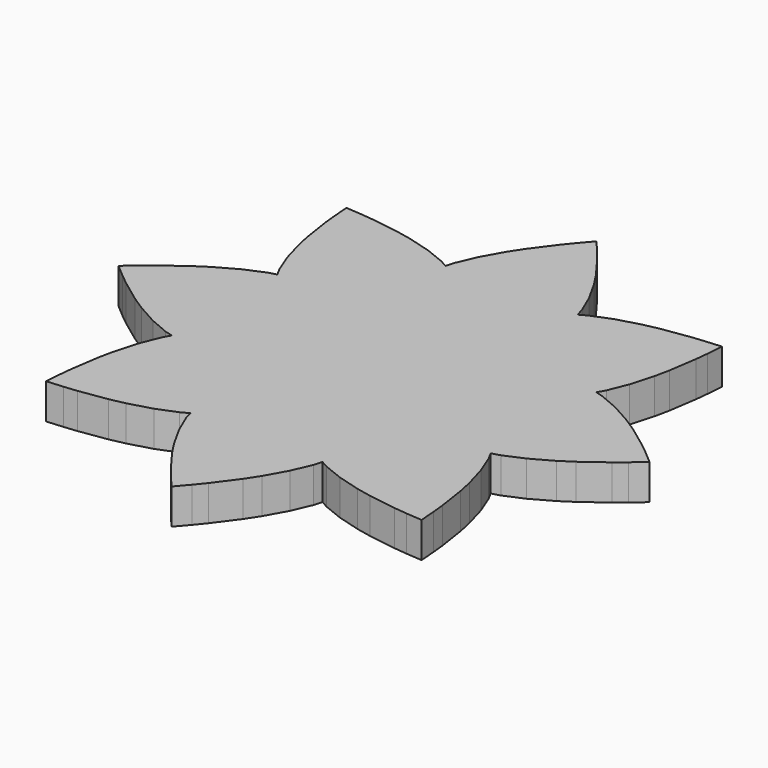
from build123d import *

# Parameters (mm, degrees)
F1_DEPTH = 6


with BuildPart() as f1:
    # F0 (on Top) → F1 (new body)
    with BuildSketch(Plane.XY):
        with BuildLine():
            ThreePointArc((11.0582894347, -1.2164948741), (11.1083098391, -0.6091613247), (11.125, 0))
            ThreePointArc((11.125, 0), (11.1083098391, 0.6091613247), (11.0582894347, 1.2164948741))
            Line((11.0582894347, 1.2164948741), (5.1512120865, 0.50045829))
            Line((5.1512120865, 0.50045829), (0, 0))
            Line((0, 0), (5.1512120865, -0.50045829))
            Line((5.1512120865, -0.50045829), (11.0582894347, -1.2164948741))
        make_face()
        with BuildLine():
            ThreePointArc((11.0582894347, 1.2164948741), (11.1083098391, 0.6091613247), (11.125, 0))
            ThreePointArc((11.125, 0), (11.1083098391, -0.6091613247), (11.0582894347, -1.2164948741))
            Line((11.0582894347, -1.2164948741), (14.5342076496, -1.8604729178))
            ThreePointArc((14.5342076496, -1.8604729178), (14.6231219501, -0.9321244087), (14.6528001242, 0))
            ThreePointArc((14.6528001242, 0), (14.6231219501, 0.9321244087), (14.5342076496, 1.8604729178))
            Line((14.5342076496, 1.8604729178), (11.0582894347, 1.2164948741))
        make_face()
        with BuildLine():
            Line((5.1512120865, 0.50045829), (11.0582894347, 1.2164948741))
            ThreePointArc((11.0582894347, 1.2164948741), (10.2781597992, 4.2573531851), (8.6795832223, 6.9591996729))
            Line((8.6795832223, 6.9591996729), (3.9963344483, 3.2885795472))
            Line((3.9963344483, 3.2885795472), (0, 0))
            Line((0, 0), (5.1512120865, 0.50045829))
        make_face()
        with BuildLine():
            ThreePointArc((8.6795832223, 6.9591996729), (10.2781597992, 4.2573531851), (11.0582894347, 1.2164948741))
            Line((11.0582894347, 1.2164948741), (14.5342076496, 1.8604729178))
            ThreePointArc((14.5342076496, 1.8604729178), (13.5374221288, 5.6073838453), (11.5927898046, 8.9616837719))
            Line((11.5927898046, 8.9616837719), (8.6795832223, 6.9591996729))
        make_face()
        with BuildLine():
            Line((14.5342076496, -1.8604729178), (11.0582894347, -1.2164948741))
            ThreePointArc((11.0582894347, -1.2164948741), (10.2781597992, -4.2573531851), (8.6795832223, -6.9591996729))
            Line((8.6795832223, -6.9591996729), (11.5927898046, -8.9616837719))
            ThreePointArc((11.5927898046, -8.9616837719), (13.5374221288, -5.6073838453), (14.5342076496, -1.8604729178))
        make_face()
        with BuildLine():
            ThreePointArc((8.6795832223, -6.9591996729), (10.2781597992, -4.2573531851), (11.0582894347, -1.2164948741))
            Line((11.0582894347, -1.2164948741), (5.1512120865, -0.50045829))
            Line((5.1512120865, -0.50045829), (0, 0))
            Line((0, 0), (3.9963344483, -3.2885795472))
            Line((3.9963344483, -3.2885795472), (8.6795832223, -6.9591996729))
        make_face()
        with BuildLine():
            Line((3.9963344483, 3.2885795472), (8.6795832223, 6.9591996729))
            ThreePointArc((8.6795832223, 6.9591996729), (7.8665629407, 7.8665629407), (6.9591996729, 8.6795832223))
            Line((6.9591996729, 8.6795832223), (3.2885795472, 3.9963344483))
            Line((3.2885795472, 3.9963344483), (0, 0))
            Line((0, 0), (3.9963344483, 3.2885795472))
        make_face()
        with BuildLine():
            ThreePointArc((6.9591996729, 8.6795832223), (7.8665629407, 7.8665629407), (8.6795832223, 6.9591996729))
            Line((8.6795832223, 6.9591996729), (11.5927898046, 8.9616837719))
            ThreePointArc((11.5927898046, 8.9616837719), (10.3610943312, 10.3610943312), (8.9616837719, 11.5927898046))
            Line((8.9616837719, 11.5927898046), (6.9591996729, 8.6795832223))
        make_face()
        with BuildLine():
            Line((15.430184363, 2.1339611713), (14.5342076496, 1.8604729178))
            ThreePointArc((14.5342076496, 1.8604729178), (14.6231219501, 0.9321244087), (14.6528001242, 0))
            ThreePointArc((14.6528001242, 0), (14.6231219501, -0.9321244087), (14.5342076496, -1.8604729178))
            Line((14.5342076496, -1.8604729178), (15.430184363, -2.1339611713))
            ThreePointArc((15.430184363, -2.1339611713), (15.124443045, 0), (15.430184363, 2.1339611713))
        make_face()
        with BuildLine():
            ThreePointArc((11.5927898046, 8.9616837719), (13.5374221288, 5.6073838453), (14.5342076496, 1.8604729178))
            Line((14.5342076496, 1.8604729178), (15.430184363, 2.1339611713))
            ThreePointArc((15.430184363, 2.1339611713), (18.8444497658, 6.5349561707), (24.3428657322, 7.4256789592))
            Line((24.3428657322, 7.4256789592), (26.2042805414, 9.6967201996))
            Line((26.2042805414, 9.6967201996), (27.0298449885, 11.1961283831))
            Line((27.0298449885, 11.1961283831), (25.3858410754, 11.6726078585))
            Line((25.3858410754, 11.6726078585), (22.4637533797, 11.9622574858))
            ThreePointArc((22.4637533797, 11.9622574858), (17.9459500402, 8.704126394), (12.419726413, 9.401849583))
            Line((12.419726413, 9.401849583), (11.5927898046, 8.9616837719))
        make_face()
        with BuildLine():
            Line((11.5927898046, -8.9616837719), (8.6795832223, -6.9591996729))
            ThreePointArc((8.6795832223, -6.9591996729), (7.8665629407, -7.8665629407), (6.9591996729, -8.6795832223))
            Line((6.9591996729, -8.6795832223), (8.9616837719, -11.5927898046))
            ThreePointArc((8.9616837719, -11.5927898046), (10.3610943312, -10.3610943312), (11.5927898046, -8.9616837719))
        make_face()
        with BuildLine():
            ThreePointArc((6.9591996729, -8.6795832223), (7.8665629407, -7.8665629407), (8.6795832223, -6.9591996729))
            Line((8.6795832223, -6.9591996729), (3.9963344483, -3.2885795472))
            Line((3.9963344483, -3.2885795472), (0, 0))
            Line((0, 0), (3.2885795472, -3.9963344483))
            Line((3.2885795472, -3.9963344483), (6.9591996729, -8.6795832223))
        make_face()
        with BuildLine():
            Line((15.430184363, -2.1339611713), (14.5342076496, -1.8604729178))
            ThreePointArc((14.5342076496, -1.8604729178), (13.5374221288, -5.6073838453), (11.5927898046, -8.9616837719))
            Line((11.5927898046, -8.9616837719), (12.419726413, -9.401849583))
            ThreePointArc((12.419726413, -9.401849583), (17.9459500402, -8.704126394), (22.4637533797, -11.9622574858))
            Line((22.4637533797, -11.9622574858), (25.3858410754, -11.6726078585))
            Line((25.3858410754, -11.6726078585), (27.0298449885, -11.1961283831))
            Line((27.0298449885, -11.1961283831), (26.2042805414, -9.6967201996))
            Line((26.2042805414, -9.6967201996), (24.3428657322, -7.4256789592))
            ThreePointArc((24.3428657322, -7.4256789592), (18.8444497658, -6.5349561707), (15.430184363, -2.1339611713))
        make_face()
        with BuildLine():
            Line((3.2885795472, 3.9963344483), (6.9591996729, 8.6795832223))
            ThreePointArc((6.9591996729, 8.6795832223), (4.2573531851, 10.2781597992), (1.2164948741, 11.0582894347))
            Line((1.2164948741, 11.0582894347), (0.50045829, 5.1512120865))
            Line((0.50045829, 5.1512120865), (0, 0))
            Line((0, 0), (3.2885795472, 3.9963344483))
        make_face()
        with BuildLine():
            ThreePointArc((1.2164948741, 11.0582894347), (4.2573531851, 10.2781597992), (6.9591996729, 8.6795832223))
            Line((6.9591996729, 8.6795832223), (8.9616837719, 11.5927898046))
            ThreePointArc((8.9616837719, 11.5927898046), (5.6073838453, 13.5374221288), (1.8604729178, 14.5342076496))
            Line((1.8604729178, 14.5342076496), (1.2164948741, 11.0582894347))
        make_face()
        with BuildLine():
            ThreePointArc((8.9616837719, 11.5927898046), (10.3610943312, 10.3610943312), (11.5927898046, 8.9616837719))
            Line((11.5927898046, 8.9616837719), (12.419726413, 9.401849583))
            ThreePointArc((12.419726413, 9.401849583), (10.6945962388, 10.6945962388), (9.401849583, 12.419726413))
            Line((9.401849583, 12.419726413), (8.9616837719, 11.5927898046))
        make_face()
        with BuildLine():
            Line((-0.50045829, 5.1512120865), (0, 0))
            Line((0, 0), (0.50045829, 5.1512120865))
            Line((0.50045829, 5.1512120865), (1.2164948741, 11.0582894347))
            ThreePointArc((1.2164948741, 11.0582894347), (0, 11.125), (-1.2164948741, 11.0582894347))
            Line((-1.2164948741, 11.0582894347), (-0.50045829, 5.1512120865))
        make_face()
        with BuildLine():
            Line((-3.9963344483, 3.2885795472), (0, 0))
            Line((0, 0), (-3.2885795472, 3.9963344483))
            Line((-3.2885795472, 3.9963344483), (-6.9591996729, 8.6795832223))
            ThreePointArc((-6.9591996729, 8.6795832223), (-7.8665629407, 7.8665629407), (-8.6795832223, 6.9591996729))
            Line((-8.6795832223, 6.9591996729), (-3.9963344483, 3.2885795472))
        make_face()
        with BuildLine():
            Line((-5.1512120865, -0.50045829), (0, 0))
            Line((0, 0), (-5.1512120865, 0.50045829))
            Line((-5.1512120865, 0.50045829), (-11.0582894347, 1.2164948741))
            ThreePointArc((-11.0582894347, 1.2164948741), (-11.125, 0), (-11.0582894347, -1.2164948741))
            Line((-11.0582894347, -1.2164948741), (-5.1512120865, -0.50045829))
        make_face()
        with BuildLine():
            Line((-3.2885795472, 3.9963344483), (0, 0))
            Line((0, 0), (-0.50045829, 5.1512120865))
            Line((-0.50045829, 5.1512120865), (-1.2164948741, 11.0582894347))
            ThreePointArc((-1.2164948741, 11.0582894347), (-4.2573531851, 10.2781597992), (-6.9591996729, 8.6795832223))
            Line((-6.9591996729, 8.6795832223), (-3.2885795472, 3.9963344483))
        make_face()
        with BuildLine():
            Line((-3.2885795472, -3.9963344483), (0, 0))
            Line((0, 0), (-3.9963344483, -3.2885795472))
            Line((-3.9963344483, -3.2885795472), (-8.6795832223, -6.9591996729))
            ThreePointArc((-8.6795832223, -6.9591996729), (-7.8665629407, -7.8665629407), (-6.9591996729, -8.6795832223))
            Line((-6.9591996729, -8.6795832223), (-3.2885795472, -3.9963344483))
        make_face()
        with BuildLine():
            Line((-5.1512120865, 0.50045829), (0, 0))
            Line((0, 0), (-3.9963344483, 3.2885795472))
            Line((-3.9963344483, 3.2885795472), (-8.6795832223, 6.9591996729))
            ThreePointArc((-8.6795832223, 6.9591996729), (-10.2781597992, 4.2573531851), (-11.0582894347, 1.2164948741))
            Line((-11.0582894347, 1.2164948741), (-5.1512120865, 0.50045829))
        make_face()
        with BuildLine():
            Line((0.50045829, -5.1512120865), (0, 0))
            Line((0, 0), (-0.50045829, -5.1512120865))
            Line((-0.50045829, -5.1512120865), (-1.2164948741, -11.0582894347))
            ThreePointArc((-1.2164948741, -11.0582894347), (0, -11.125), (1.2164948741, -11.0582894347))
            Line((1.2164948741, -11.0582894347), (0.50045829, -5.1512120865))
        make_face()
        with BuildLine():
            Line((-3.9963344483, -3.2885795472), (0, 0))
            Line((0, 0), (-5.1512120865, -0.50045829))
            Line((-5.1512120865, -0.50045829), (-11.0582894347, -1.2164948741))
            ThreePointArc((-11.0582894347, -1.2164948741), (-10.2781597992, -4.2573531851), (-8.6795832223, -6.9591996729))
            Line((-8.6795832223, -6.9591996729), (-3.9963344483, -3.2885795472))
        make_face()
        with BuildLine():
            Line((-0.50045829, -5.1512120865), (0, 0))
            Line((0, 0), (-3.2885795472, -3.9963344483))
            Line((-3.2885795472, -3.9963344483), (-6.9591996729, -8.6795832223))
            ThreePointArc((-6.9591996729, -8.6795832223), (-4.2573531851, -10.2781597992), (-1.2164948741, -11.0582894347))
            Line((-1.2164948741, -11.0582894347), (-0.50045829, -5.1512120865))
        make_face()
        with BuildLine():
            Line((3.2885795472, -3.9963344483), (0, 0))
            Line((0, 0), (0.50045829, -5.1512120865))
            Line((0.50045829, -5.1512120865), (1.2164948741, -11.0582894347))
            ThreePointArc((1.2164948741, -11.0582894347), (4.2573531851, -10.2781597992), (6.9591996729, -8.6795832223))
            Line((6.9591996729, -8.6795832223), (3.2885795472, -3.9963344483))
        make_face()
        with BuildLine():
            Line((18.2448972854, 2.9931251538), (15.430184363, 2.1339611713))
            ThreePointArc((15.430184363, 2.1339611713), (15.124443045, 0), (15.430184363, -2.1339611713))
            Line((15.430184363, -2.1339611713), (18.2448972854, -2.9931251538))
            Line((18.2448972854, -2.9931251538), (20.6460986755, -4.1929594678))
            Line((20.6460986755, -4.1929594678), (23.4293033696, -6.311076351))
            Line((23.4293033696, -6.311076351), (24.3428657322, -7.4256789592))
            ThreePointArc((24.3428657322, -7.4256789592), (28.6430582725, -4.767598325), (30.324443045, 0))
            ThreePointArc((30.324443045, 0), (28.6430582725, 4.767598325), (24.3428657322, 7.4256789592))
            Line((24.3428657322, 7.4256789592), (23.4293033696, 6.311076351))
            Line((23.4293033696, 6.311076351), (20.6460986755, 4.1929594678))
            Line((20.6460986755, 4.1929594678), (18.2448972854, 2.9931251538))
        make_face()
        with BuildLine():
            ThreePointArc((24.3428657322, 7.4256789592), (18.8444497658, 6.5349561707), (15.430184363, 2.1339611713))
            Line((15.430184363, 2.1339611713), (18.2448972854, 2.9931251538))
            Line((18.2448972854, 2.9931251538), (20.6460986755, 4.1929594678))
            Line((20.6460986755, 4.1929594678), (23.4293033696, 6.311076351))
            Line((23.4293033696, 6.311076351), (24.3428657322, 7.4256789592))
        make_face()
        with BuildLine():
            Line((8.9616837719, -11.5927898046), (6.9591996729, -8.6795832223))
            ThreePointArc((6.9591996729, -8.6795832223), (4.2573531851, -10.2781597992), (1.2164948741, -11.0582894347))
            Line((1.2164948741, -11.0582894347), (1.8604729178, -14.5342076496))
            ThreePointArc((1.8604729178, -14.5342076496), (5.6073838453, -13.5374221288), (8.9616837719, -11.5927898046))
        make_face()
        with BuildLine():
            Line((12.419726413, -9.401849583), (11.5927898046, -8.9616837719))
            ThreePointArc((11.5927898046, -8.9616837719), (10.3610943312, -10.3610943312), (8.9616837719, -11.5927898046))
            Line((8.9616837719, -11.5927898046), (9.401849583, -12.419726413))
            ThreePointArc((9.401849583, -12.419726413), (10.6945962388, -10.6945962388), (12.419726413, -9.401849583))
        make_face()
        with BuildLine():
            Line((18.2448972854, -2.9931251538), (15.430184363, -2.1339611713))
            ThreePointArc((15.430184363, -2.1339611713), (18.8444497658, -6.5349561707), (24.3428657322, -7.4256789592))
            Line((24.3428657322, -7.4256789592), (23.4293033696, -6.311076351))
            Line((23.4293033696, -6.311076351), (20.6460986755, -4.1929594678))
            Line((20.6460986755, -4.1929594678), (18.2448972854, -2.9931251538))
        make_face()
        with BuildLine():
            ThreePointArc((-1.2164948741, 11.0582894347), (0, 11.125), (1.2164948741, 11.0582894347))
            Line((1.2164948741, 11.0582894347), (1.8604729178, 14.5342076496))
            ThreePointArc((1.8604729178, 14.5342076496), (0, 14.6528001242), (-1.8604729178, 14.5342076496))
            Line((-1.8604729178, 14.5342076496), (-1.2164948741, 11.0582894347))
        make_face()
        with BuildLine():
            ThreePointArc((1.8604729178, 14.5342076496), (5.6073838453, 13.5374221288), (8.9616837719, 11.5927898046))
            Line((8.9616837719, 11.5927898046), (9.401849583, 12.419726413))
            ThreePointArc((9.401849583, 12.419726413), (8.704126394, 17.9459500402), (11.9622574858, 22.4637533797))
            Line((11.9622574858, 22.4637533797), (11.6726078585, 25.3858410754))
            Line((11.6726078585, 25.3858410754), (11.1961283831, 27.0298449885))
            Line((11.1961283831, 27.0298449885), (9.6967201996, 26.2042805414))
            Line((9.6967201996, 26.2042805414), (7.4256789592, 24.3428657322))
            ThreePointArc((7.4256789592, 24.3428657322), (7.5562940682, 23.538334902), (7.6, 22.724443045))
            ThreePointArc((7.6, 22.724443045), (6.0818625807, 18.1669275432), (2.1339611713, 15.430184363))
            Line((2.1339611713, 15.430184363), (1.8604729178, 14.5342076496))
        make_face()
        with BuildLine():
            ThreePointArc((9.401849583, 12.419726413), (10.6945962388, 10.6945962388), (12.419726413, 9.401849583))
            Line((12.419726413, 9.401849583), (15.0175496857, 10.7846314994))
            Line((15.0175496857, 10.7846314994), (17.5638664514, 11.6341263056))
            Line((17.5638664514, 11.6341263056), (21.0296241755, 12.1044144067))
            Line((21.0296241755, 12.1044144067), (22.4637533797, 11.9622574858))
            ThreePointArc((22.4637533797, 11.9622574858), (23.3611761365, 13.9288772542), (23.6686077758, 16.0686077758))
            ThreePointArc((23.6686077758, 16.0686077758), (19.7122143542, 22.7382502776), (11.9622574858, 22.4637533797))
            Line((11.9622574858, 22.4637533797), (12.1044144067, 21.0296241755))
            Line((12.1044144067, 21.0296241755), (11.6341263056, 17.5638664514))
            Line((11.6341263056, 17.5638664514), (10.7846314994, 15.0175496857))
            Line((10.7846314994, 15.0175496857), (9.401849583, 12.419726413))
        make_face()
        with BuildLine():
            Line((15.0175496857, 10.7846314994), (12.419726413, 9.401849583))
            ThreePointArc((12.419726413, 9.401849583), (17.9459500402, 8.704126394), (22.4637533797, 11.9622574858))
            Line((22.4637533797, 11.9622574858), (21.0296241755, 12.1044144067))
            Line((21.0296241755, 12.1044144067), (17.5638664514, 11.6341263056))
            Line((17.5638664514, 11.6341263056), (15.0175496857, 10.7846314994))
        make_face()
        with BuildLine():
            Line((26.2042805414, 9.6967201996), (24.3428657322, 7.4256789592))
            ThreePointArc((24.3428657322, 7.4256789592), (28.6430582725, 4.767598325), (30.324443045, 0))
            ThreePointArc((30.324443045, 0), (28.6430582725, -4.767598325), (24.3428657322, -7.4256789592))
            Line((24.3428657322, -7.4256789592), (26.2042805414, -9.6967201996))
            Line((26.2042805414, -9.6967201996), (27.0298449885, -11.1961283831))
            Line((27.0298449885, -11.1961283831), (28.4310324357, -10.7900240822))
            Line((28.4310324357, -10.7900240822), (31.6744188466, -9.3996720824))
            Line((31.6744188466, -9.3996720824), (35.1670132617, -7.4534773141))
            Line((35.1670132617, -7.4534773141), (37.3724974487, -6.0145420413))
            Line((37.3724974487, -6.0145420413), (41.1990018918, -3.1819616895))
            Line((41.1990018918, -3.1819616895), (42.9000411602, -1.7999774681))
            Line((42.9000411602, -1.7999774681), (45, 0))
            Line((45, 0), (42.9000411602, 1.7999774681))
            Line((42.9000411602, 1.7999774681), (41.1990018918, 3.1819616895))
            Line((41.1990018918, 3.1819616895), (37.3724974487, 6.0145420413))
            Line((37.3724974487, 6.0145420413), (35.1670132617, 7.4534773141))
            Line((35.1670132617, 7.4534773141), (31.6744188466, 9.3996720824))
            Line((31.6744188466, 9.3996720824), (28.4310324357, 10.7900240822))
            Line((28.4310324357, 10.7900240822), (27.0298449885, 11.1961283831))
            Line((27.0298449885, 11.1961283831), (26.2042805414, 9.6967201996))
        make_face()
        with BuildLine():
            Line((1.8604729178, -14.5342076496), (1.2164948741, -11.0582894347))
            ThreePointArc((1.2164948741, -11.0582894347), (0, -11.125), (-1.2164948741, -11.0582894347))
            Line((-1.2164948741, -11.0582894347), (-1.8604729178, -14.5342076496))
            ThreePointArc((-1.8604729178, -14.5342076496), (0, -14.6528001242), (1.8604729178, -14.5342076496))
        make_face()
        with BuildLine():
            Line((9.401849583, -12.419726413), (8.9616837719, -11.5927898046))
            ThreePointArc((8.9616837719, -11.5927898046), (5.6073838453, -13.5374221288), (1.8604729178, -14.5342076496))
            Line((1.8604729178, -14.5342076496), (2.1339611713, -15.430184363))
            ThreePointArc((2.1339611713, -15.430184363), (6.0818625807, -18.1669275432), (7.6, -22.724443045))
            ThreePointArc((7.6, -22.724443045), (7.5562940682, -23.538334902), (7.4256789592, -24.3428657322))
            Line((7.4256789592, -24.3428657322), (9.6967201996, -26.2042805414))
            Line((9.6967201996, -26.2042805414), (11.1961283831, -27.0298449885))
            Line((11.1961283831, -27.0298449885), (11.6726078585, -25.3858410754))
            Line((11.6726078585, -25.3858410754), (11.9622574858, -22.4637533797))
            ThreePointArc((11.9622574858, -22.4637533797), (8.704126394, -17.9459500402), (9.401849583, -12.419726413))
        make_face()
        with BuildLine():
            ThreePointArc((22.4637533797, -11.9622574858), (17.9459500402, -8.704126394), (12.419726413, -9.401849583))
            Line((12.419726413, -9.401849583), (15.0175496857, -10.7846314994))
            Line((15.0175496857, -10.7846314994), (17.5638664514, -11.6341263056))
            Line((17.5638664514, -11.6341263056), (21.0296241755, -12.1044144067))
            Line((21.0296241755, -12.1044144067), (22.4637533797, -11.9622574858))
        make_face()
        with BuildLine():
            Line((15.0175496857, -10.7846314994), (12.419726413, -9.401849583))
            ThreePointArc((12.419726413, -9.401849583), (10.6945962388, -10.6945962388), (9.401849583, -12.419726413))
            Line((9.401849583, -12.419726413), (10.7846314994, -15.0175496857))
            Line((10.7846314994, -15.0175496857), (11.6341263056, -17.5638664514))
            Line((11.6341263056, -17.5638664514), (12.1044144067, -21.0296241755))
            Line((12.1044144067, -21.0296241755), (11.9622574858, -22.4637533797))
            ThreePointArc((11.9622574858, -22.4637533797), (19.7122143542, -22.7382502776), (23.6686077758, -16.0686077758))
            ThreePointArc((23.6686077758, -16.0686077758), (23.3611761365, -13.9288772542), (22.4637533797, -11.9622574858))
            Line((22.4637533797, -11.9622574858), (21.0296241755, -12.1044144067))
            Line((21.0296241755, -12.1044144067), (17.5638664514, -11.6341263056))
            Line((17.5638664514, -11.6341263056), (15.0175496857, -10.7846314994))
        make_face()
        with BuildLine():
            ThreePointArc((-6.9591996729, 8.6795832223), (-4.2573531851, 10.2781597992), (-1.2164948741, 11.0582894347))
            Line((-1.2164948741, 11.0582894347), (-1.8604729178, 14.5342076496))
            ThreePointArc((-1.8604729178, 14.5342076496), (-5.6073838453, 13.5374221288), (-8.9616837719, 11.5927898046))
            Line((-8.9616837719, 11.5927898046), (-6.9591996729, 8.6795832223))
        make_face()
        with BuildLine():
            ThreePointArc((-1.8604729178, 14.5342076496), (0, 14.6528001242), (1.8604729178, 14.5342076496))
            Line((1.8604729178, 14.5342076496), (2.1339611713, 15.430184363))
            ThreePointArc((2.1339611713, 15.430184363), (0, 15.124443045), (-2.1339611713, 15.430184363))
            Line((-2.1339611713, 15.430184363), (-1.8604729178, 14.5342076496))
        make_face()
        with BuildLine():
            ThreePointArc((11.9622574858, 22.4637533797), (8.704126394, 17.9459500402), (9.401849583, 12.419726413))
            Line((9.401849583, 12.419726413), (10.7846314994, 15.0175496857))
            Line((10.7846314994, 15.0175496857), (11.6341263056, 17.5638664514))
            Line((11.6341263056, 17.5638664514), (12.1044144067, 21.0296241755))
            Line((12.1044144067, 21.0296241755), (11.9622574858, 22.4637533797))
        make_face()
        with BuildLine():
            ThreePointArc((23.6686077758, 16.0686077758), (23.3611761365, 13.9288772542), (22.4637533797, 11.9622574858))
            Line((22.4637533797, 11.9622574858), (25.3858410754, 11.6726078585))
            Line((25.3858410754, 11.6726078585), (27.0298449885, 11.1961283831))
            Line((27.0298449885, 11.1961283831), (27.7334750291, 12.4740766338))
            Line((27.7334750291, 12.4740766338), (29.043768227, 15.7506244862))
            Line((29.043768227, 15.7506244862), (30.1372379036, 19.5964291992))
            Line((30.1372379036, 19.5964291992), (30.679269839, 22.1734229128))
            Line((30.679269839, 22.1734229128), (31.382080304, 26.8821069277))
            Line((31.382080304, 26.8821069277), (31.6076862912, 29.0621337438))
            Line((31.6076862912, 29.0621337438), (31.8198051534, 31.8198051534))
            Line((31.8198051534, 31.8198051534), (29.0621337438, 31.6076862912))
            Line((29.0621337438, 31.6076862912), (26.8821069277, 31.382080304))
            Line((26.8821069277, 31.382080304), (22.1734229128, 30.679269839))
            Line((22.1734229128, 30.679269839), (19.5964291992, 30.1372379036))
            Line((19.5964291992, 30.1372379036), (15.7506244862, 29.043768227))
            Line((15.7506244862, 29.043768227), (12.4740766338, 27.7334750291))
            Line((12.4740766338, 27.7334750291), (11.1961283831, 27.0298449885))
            Line((11.1961283831, 27.0298449885), (11.6726078585, 25.3858410754))
            Line((11.6726078585, 25.3858410754), (11.9622574858, 22.4637533797))
            ThreePointArc((11.9622574858, 22.4637533797), (19.7122143542, 22.7382502776), (23.6686077758, 16.0686077758))
        make_face()
        with BuildLine():
            ThreePointArc((-8.6795832223, 6.9591996729), (-7.8665629407, 7.8665629407), (-6.9591996729, 8.6795832223))
            Line((-6.9591996729, 8.6795832223), (-8.9616837719, 11.5927898046))
            ThreePointArc((-8.9616837719, 11.5927898046), (-10.3610943312, 10.3610943312), (-11.5927898046, 8.9616837719))
            Line((-11.5927898046, 8.9616837719), (-8.6795832223, 6.9591996729))
        make_face()
        with BuildLine():
            Line((-14.5342076496, 1.8604729178), (-11.0582894347, 1.2164948741))
            ThreePointArc((-11.0582894347, 1.2164948741), (-10.2781597992, 4.2573531851), (-8.6795832223, 6.9591996729))
            Line((-8.6795832223, 6.9591996729), (-11.5927898046, 8.9616837719))
            ThreePointArc((-11.5927898046, 8.9616837719), (-13.5374221288, 5.6073838453), (-14.5342076496, 1.8604729178))
        make_face()
        with BuildLine():
            ThreePointArc((-11.0582894347, -1.2164948741), (-11.125, 0), (-11.0582894347, 1.2164948741))
            Line((-11.0582894347, 1.2164948741), (-14.5342076496, 1.8604729178))
            ThreePointArc((-14.5342076496, 1.8604729178), (-14.6528001242, 0), (-14.5342076496, -1.8604729178))
            Line((-14.5342076496, -1.8604729178), (-11.0582894347, -1.2164948741))
        make_face()
        with BuildLine():
            Line((-11.5927898046, -8.9616837719), (-8.6795832223, -6.9591996729))
            ThreePointArc((-8.6795832223, -6.9591996729), (-10.2781597992, -4.2573531851), (-11.0582894347, -1.2164948741))
            Line((-11.0582894347, -1.2164948741), (-14.5342076496, -1.8604729178))
            ThreePointArc((-14.5342076496, -1.8604729178), (-13.5374221288, -5.6073838453), (-11.5927898046, -8.9616837719))
        make_face()
        with BuildLine():
            ThreePointArc((-6.9591996729, -8.6795832223), (-7.8665629407, -7.8665629407), (-8.6795832223, -6.9591996729))
            Line((-8.6795832223, -6.9591996729), (-11.5927898046, -8.9616837719))
            ThreePointArc((-11.5927898046, -8.9616837719), (-10.3610943312, -10.3610943312), (-8.9616837719, -11.5927898046))
            Line((-8.9616837719, -11.5927898046), (-6.9591996729, -8.6795832223))
        make_face()
        with BuildLine():
            Line((-1.8604729178, -14.5342076496), (-1.2164948741, -11.0582894347))
            ThreePointArc((-1.2164948741, -11.0582894347), (-4.2573531851, -10.2781597992), (-6.9591996729, -8.6795832223))
            Line((-6.9591996729, -8.6795832223), (-8.9616837719, -11.5927898046))
            ThreePointArc((-8.9616837719, -11.5927898046), (-5.6073838453, -13.5374221288), (-1.8604729178, -14.5342076496))
        make_face()
        with BuildLine():
            Line((2.1339611713, -15.430184363), (1.8604729178, -14.5342076496))
            ThreePointArc((1.8604729178, -14.5342076496), (0, -14.6528001242), (-1.8604729178, -14.5342076496))
            Line((-1.8604729178, -14.5342076496), (-2.1339611713, -15.430184363))
            ThreePointArc((-2.1339611713, -15.430184363), (0, -15.124443045), (2.1339611713, -15.430184363))
        make_face()
        with BuildLine():
            Line((10.7846314994, -15.0175496857), (9.401849583, -12.419726413))
            ThreePointArc((9.401849583, -12.419726413), (8.704126394, -17.9459500402), (11.9622574858, -22.4637533797))
            Line((11.9622574858, -22.4637533797), (12.1044144067, -21.0296241755))
            Line((12.1044144067, -21.0296241755), (11.6341263056, -17.5638664514))
            Line((11.6341263056, -17.5638664514), (10.7846314994, -15.0175496857))
        make_face()
        with BuildLine():
            Line((25.3858410754, -11.6726078585), (22.4637533797, -11.9622574858))
            ThreePointArc((22.4637533797, -11.9622574858), (23.3611761365, -13.9288772542), (23.6686077758, -16.0686077758))
            ThreePointArc((23.6686077758, -16.0686077758), (19.7122143542, -22.7382502776), (11.9622574858, -22.4637533797))
            Line((11.9622574858, -22.4637533797), (11.6726078585, -25.3858410754))
            Line((11.6726078585, -25.3858410754), (11.1961283831, -27.0298449885))
            Line((11.1961283831, -27.0298449885), (12.4740766338, -27.7334750291))
            Line((12.4740766338, -27.7334750291), (15.7506244862, -29.043768227))
            Line((15.7506244862, -29.043768227), (19.5964291992, -30.1372379036))
            Line((19.5964291992, -30.1372379036), (22.1734229128, -30.679269839))
            Line((22.1734229128, -30.679269839), (26.8821069277, -31.382080304))
            Line((26.8821069277, -31.382080304), (29.0621337438, -31.6076862912))
            Line((29.0621337438, -31.6076862912), (31.8198051534, -31.8198051534))
            Line((31.8198051534, -31.8198051534), (31.6076862912, -29.0621337438))
            Line((31.6076862912, -29.0621337438), (31.382080304, -26.8821069277))
            Line((31.382080304, -26.8821069277), (30.679269839, -22.1734229128))
            Line((30.679269839, -22.1734229128), (30.1372379036, -19.5964291992))
            Line((30.1372379036, -19.5964291992), (29.043768227, -15.7506244862))
            Line((29.043768227, -15.7506244862), (27.7334750291, -12.4740766338))
            Line((27.7334750291, -12.4740766338), (27.0298449885, -11.1961283831))
            Line((27.0298449885, -11.1961283831), (25.3858410754, -11.6726078585))
        make_face()
        with BuildLine():
            ThreePointArc((-8.9616837719, 11.5927898046), (-5.6073838453, 13.5374221288), (-1.8604729178, 14.5342076496))
            Line((-1.8604729178, 14.5342076496), (-2.1339611713, 15.430184363))
            ThreePointArc((-2.1339611713, 15.430184363), (-6.5349561707, 18.8444497658), (-7.4256789592, 24.3428657322))
            Line((-7.4256789592, 24.3428657322), (-9.6967201996, 26.2042805414))
            Line((-9.6967201996, 26.2042805414), (-11.1961283831, 27.0298449885))
            Line((-11.1961283831, 27.0298449885), (-11.6726078585, 25.3858410754))
            Line((-11.6726078585, 25.3858410754), (-11.9622574858, 22.4637533797))
            ThreePointArc((-11.9622574858, 22.4637533797), (-9.398965274, 19.7122143542), (-8.4686077758, 16.0686077758))
            ThreePointArc((-8.4686077758, 16.0686077758), (-8.7056137426, 14.1854405321), (-9.401849583, 12.419726413))
            Line((-9.401849583, 12.419726413), (-8.9616837719, 11.5927898046))
        make_face()
        with BuildLine():
            ThreePointArc((-2.1339611713, 15.430184363), (0, 15.124443045), (2.1339611713, 15.430184363))
            Line((2.1339611713, 15.430184363), (2.9931251538, 18.2448972854))
            Line((2.9931251538, 18.2448972854), (4.1929594678, 20.6460986755))
            Line((4.1929594678, 20.6460986755), (6.311076351, 23.4293033696))
            Line((6.311076351, 23.4293033696), (7.4256789592, 24.3428657322))
            ThreePointArc((7.4256789592, 24.3428657322), (0, 30.324443045), (-7.4256789592, 24.3428657322))
            Line((-7.4256789592, 24.3428657322), (-6.311076351, 23.4293033696))
            Line((-6.311076351, 23.4293033696), (-4.1929594678, 20.6460986755))
            Line((-4.1929594678, 20.6460986755), (-2.9931251538, 18.2448972854))
            Line((-2.9931251538, 18.2448972854), (-2.1339611713, 15.430184363))
        make_face()
        with BuildLine():
            Line((2.9931251538, 18.2448972854), (2.1339611713, 15.430184363))
            ThreePointArc((2.1339611713, 15.430184363), (6.0818625807, 18.1669275432), (7.6, 22.724443045))
            ThreePointArc((7.6, 22.724443045), (7.5562940682, 23.538334902), (7.4256789592, 24.3428657322))
            Line((7.4256789592, 24.3428657322), (6.311076351, 23.4293033696))
            Line((6.311076351, 23.4293033696), (4.1929594678, 20.6460986755))
            Line((4.1929594678, 20.6460986755), (2.9931251538, 18.2448972854))
        make_face()
        with BuildLine():
            ThreePointArc((-11.5927898046, 8.9616837719), (-10.3610943312, 10.3610943312), (-8.9616837719, 11.5927898046))
            Line((-8.9616837719, 11.5927898046), (-9.401849583, 12.419726413))
            ThreePointArc((-9.401849583, 12.419726413), (-10.6945962388, 10.6945962388), (-12.419726413, 9.401849583))
            Line((-12.419726413, 9.401849583), (-11.5927898046, 8.9616837719))
        make_face()
        with BuildLine():
            Line((-15.430184363, 2.1339611713), (-14.5342076496, 1.8604729178))
            ThreePointArc((-14.5342076496, 1.8604729178), (-13.5374221288, 5.6073838453), (-11.5927898046, 8.9616837719))
            Line((-11.5927898046, 8.9616837719), (-12.419726413, 9.401849583))
            ThreePointArc((-12.419726413, 9.401849583), (-17.9459500402, 8.704126394), (-22.4637533797, 11.9622574858))
            Line((-22.4637533797, 11.9622574858), (-25.3858410754, 11.6726078585))
            Line((-25.3858410754, 11.6726078585), (-27.0298449885, 11.1961283831))
            Line((-27.0298449885, 11.1961283831), (-26.2042805414, 9.6967201996))
            Line((-26.2042805414, 9.6967201996), (-24.3428657322, 7.4256789592))
            ThreePointArc((-24.3428657322, 7.4256789592), (-18.8444497658, 6.5349561707), (-15.430184363, 2.1339611713))
        make_face()
        with BuildLine():
            ThreePointArc((-14.5342076496, -1.8604729178), (-14.6528001242, 0), (-14.5342076496, 1.8604729178))
            Line((-14.5342076496, 1.8604729178), (-15.430184363, 2.1339611713))
            ThreePointArc((-15.430184363, 2.1339611713), (-15.2012666552, 1.0778761564), (-15.124443045, 0))
            ThreePointArc((-15.124443045, 0), (-15.2012666552, -1.0778761564), (-15.430184363, -2.1339611713))
            Line((-15.430184363, -2.1339611713), (-14.5342076496, -1.8604729178))
        make_face()
        with BuildLine():
            Line((-12.419726413, -9.401849583), (-11.5927898046, -8.9616837719))
            ThreePointArc((-11.5927898046, -8.9616837719), (-13.5374221288, -5.6073838453), (-14.5342076496, -1.8604729178))
            Line((-14.5342076496, -1.8604729178), (-15.430184363, -2.1339611713))
            ThreePointArc((-15.430184363, -2.1339611713), (-18.8444497658, -6.5349561707), (-24.3428657322, -7.4256789592))
            Line((-24.3428657322, -7.4256789592), (-26.2042805414, -9.6967201996))
            Line((-26.2042805414, -9.6967201996), (-27.0298449885, -11.1961283831))
            Line((-27.0298449885, -11.1961283831), (-25.3858410754, -11.6726078585))
            Line((-25.3858410754, -11.6726078585), (-22.4637533797, -11.9622574858))
            ThreePointArc((-22.4637533797, -11.9622574858), (-17.9459500402, -8.704126394), (-12.419726413, -9.401849583))
        make_face()
        with BuildLine():
            ThreePointArc((-8.9616837719, -11.5927898046), (-10.3610943312, -10.3610943312), (-11.5927898046, -8.9616837719))
            Line((-11.5927898046, -8.9616837719), (-12.419726413, -9.401849583))
            ThreePointArc((-12.419726413, -9.401849583), (-10.6945962388, -10.6945962388), (-9.401849583, -12.419726413))
            Line((-9.401849583, -12.419726413), (-8.9616837719, -11.5927898046))
        make_face()
        with BuildLine():
            Line((-2.1339611713, -15.430184363), (-1.8604729178, -14.5342076496))
            ThreePointArc((-1.8604729178, -14.5342076496), (-5.6073838453, -13.5374221288), (-8.9616837719, -11.5927898046))
            Line((-8.9616837719, -11.5927898046), (-9.401849583, -12.419726413))
            ThreePointArc((-9.401849583, -12.419726413), (-8.7056137426, -14.1854405321), (-8.4686077758, -16.0686077758))
            ThreePointArc((-8.4686077758, -16.0686077758), (-9.398965274, -19.7122143542), (-11.9622574858, -22.4637533797))
            Line((-11.9622574858, -22.4637533797), (-11.6726078585, -25.3858410754))
            Line((-11.6726078585, -25.3858410754), (-11.1961283831, -27.0298449885))
            Line((-11.1961283831, -27.0298449885), (-9.6967201996, -26.2042805414))
            Line((-9.6967201996, -26.2042805414), (-7.4256789592, -24.3428657322))
            ThreePointArc((-7.4256789592, -24.3428657322), (-6.5349561707, -18.8444497658), (-2.1339611713, -15.430184363))
        make_face()
        with BuildLine():
            Line((2.9931251538, -18.2448972854), (2.1339611713, -15.430184363))
            ThreePointArc((2.1339611713, -15.430184363), (0, -15.124443045), (-2.1339611713, -15.430184363))
            Line((-2.1339611713, -15.430184363), (-2.9931251538, -18.2448972854))
            Line((-2.9931251538, -18.2448972854), (-4.1929594678, -20.6460986755))
            Line((-4.1929594678, -20.6460986755), (-6.311076351, -23.4293033696))
            Line((-6.311076351, -23.4293033696), (-7.4256789592, -24.3428657322))
            ThreePointArc((-7.4256789592, -24.3428657322), (0, -30.324443045), (7.4256789592, -24.3428657322))
            Line((7.4256789592, -24.3428657322), (6.311076351, -23.4293033696))
            Line((6.311076351, -23.4293033696), (4.1929594678, -20.6460986755))
            Line((4.1929594678, -20.6460986755), (2.9931251538, -18.2448972854))
        make_face()
        with BuildLine():
            ThreePointArc((7.6, -22.724443045), (6.0818625807, -18.1669275432), (2.1339611713, -15.430184363))
            Line((2.1339611713, -15.430184363), (2.9931251538, -18.2448972854))
            Line((2.9931251538, -18.2448972854), (4.1929594678, -20.6460986755))
            Line((4.1929594678, -20.6460986755), (6.311076351, -23.4293033696))
            Line((6.311076351, -23.4293033696), (7.4256789592, -24.3428657322))
            ThreePointArc((7.4256789592, -24.3428657322), (7.5562940682, -23.538334902), (7.6, -22.724443045))
        make_face()
        with BuildLine():
            ThreePointArc((-7.4256789592, 24.3428657322), (-6.5349561707, 18.8444497658), (-2.1339611713, 15.430184363))
            Line((-2.1339611713, 15.430184363), (-2.9931251538, 18.2448972854))
            Line((-2.9931251538, 18.2448972854), (-4.1929594678, 20.6460986755))
            Line((-4.1929594678, 20.6460986755), (-6.311076351, 23.4293033696))
            Line((-6.311076351, 23.4293033696), (-7.4256789592, 24.3428657322))
        make_face()
        with BuildLine():
            ThreePointArc((-12.419726413, 9.401849583), (-10.6945962388, 10.6945962388), (-9.401849583, 12.419726413))
            Line((-9.401849583, 12.419726413), (-10.7846314994, 15.0175496857))
            Line((-10.7846314994, 15.0175496857), (-11.6341263056, 17.5638664514))
            Line((-11.6341263056, 17.5638664514), (-12.1044144067, 21.0296241755))
            Line((-12.1044144067, 21.0296241755), (-11.9622574858, 22.4637533797))
            ThreePointArc((-11.9622574858, 22.4637533797), (-21.4426193128, 21.4426193128), (-22.4637533797, 11.9622574858))
            Line((-22.4637533797, 11.9622574858), (-21.0296241755, 12.1044144067))
            Line((-21.0296241755, 12.1044144067), (-17.5638664514, 11.6341263056))
            Line((-17.5638664514, 11.6341263056), (-15.0175496857, 10.7846314994))
            Line((-15.0175496857, 10.7846314994), (-12.419726413, 9.401849583))
        make_face()
        with BuildLine():
            Line((-10.7846314994, 15.0175496857), (-9.401849583, 12.419726413))
            ThreePointArc((-9.401849583, 12.419726413), (-8.7056137426, 14.1854405321), (-8.4686077758, 16.0686077758))
            ThreePointArc((-8.4686077758, 16.0686077758), (-9.398965274, 19.7122143542), (-11.9622574858, 22.4637533797))
            Line((-11.9622574858, 22.4637533797), (-12.1044144067, 21.0296241755))
            Line((-12.1044144067, 21.0296241755), (-11.6341263056, 17.5638664514))
            Line((-11.6341263056, 17.5638664514), (-10.7846314994, 15.0175496857))
        make_face()
        with BuildLine():
            ThreePointArc((-15.124443045, 0), (-15.2012666552, 1.0778761564), (-15.430184363, 2.1339611713))
            Line((-15.430184363, 2.1339611713), (-18.2448972854, 2.9931251538))
            Line((-18.2448972854, 2.9931251538), (-20.6460986755, 4.1929594678))
            Line((-20.6460986755, 4.1929594678), (-23.4293033696, 6.311076351))
            Line((-23.4293033696, 6.311076351), (-24.3428657322, 7.4256789592))
            ThreePointArc((-24.3428657322, 7.4256789592), (-30.324443045, 0), (-24.3428657322, -7.4256789592))
            Line((-24.3428657322, -7.4256789592), (-23.4293033696, -6.311076351))
            Line((-23.4293033696, -6.311076351), (-20.6460986755, -4.1929594678))
            Line((-20.6460986755, -4.1929594678), (-18.2448972854, -2.9931251538))
            Line((-18.2448972854, -2.9931251538), (-15.430184363, -2.1339611713))
            ThreePointArc((-15.430184363, -2.1339611713), (-15.2012666552, -1.0778761564), (-15.124443045, 0))
        make_face()
        with BuildLine():
            Line((-18.2448972854, 2.9931251538), (-15.430184363, 2.1339611713))
            ThreePointArc((-15.430184363, 2.1339611713), (-18.8444497658, 6.5349561707), (-24.3428657322, 7.4256789592))
            Line((-24.3428657322, 7.4256789592), (-23.4293033696, 6.311076351))
            Line((-23.4293033696, 6.311076351), (-20.6460986755, 4.1929594678))
            Line((-20.6460986755, 4.1929594678), (-18.2448972854, 2.9931251538))
        make_face()
        with BuildLine():
            ThreePointArc((-9.401849583, -12.419726413), (-10.6945962388, -10.6945962388), (-12.419726413, -9.401849583))
            Line((-12.419726413, -9.401849583), (-15.0175496857, -10.7846314994))
            Line((-15.0175496857, -10.7846314994), (-17.5638664514, -11.6341263056))
            Line((-17.5638664514, -11.6341263056), (-21.0296241755, -12.1044144067))
            Line((-21.0296241755, -12.1044144067), (-22.4637533797, -11.9622574858))
            ThreePointArc((-22.4637533797, -11.9622574858), (-21.4426193128, -21.4426193128), (-11.9622574858, -22.4637533797))
            Line((-11.9622574858, -22.4637533797), (-12.1044144067, -21.0296241755))
            Line((-12.1044144067, -21.0296241755), (-11.6341263056, -17.5638664514))
            Line((-11.6341263056, -17.5638664514), (-10.7846314994, -15.0175496857))
            Line((-10.7846314994, -15.0175496857), (-9.401849583, -12.419726413))
        make_face()
        with BuildLine():
            Line((-15.0175496857, -10.7846314994), (-12.419726413, -9.401849583))
            ThreePointArc((-12.419726413, -9.401849583), (-17.9459500402, -8.704126394), (-22.4637533797, -11.9622574858))
            Line((-22.4637533797, -11.9622574858), (-21.0296241755, -12.1044144067))
            Line((-21.0296241755, -12.1044144067), (-17.5638664514, -11.6341263056))
            Line((-17.5638664514, -11.6341263056), (-15.0175496857, -10.7846314994))
        make_face()
        with BuildLine():
            ThreePointArc((-22.4637533797, 11.9622574858), (-17.9459500402, 8.704126394), (-12.419726413, 9.401849583))
            Line((-12.419726413, 9.401849583), (-15.0175496857, 10.7846314994))
            Line((-15.0175496857, 10.7846314994), (-17.5638664514, 11.6341263056))
            Line((-17.5638664514, 11.6341263056), (-21.0296241755, 12.1044144067))
            Line((-21.0296241755, 12.1044144067), (-22.4637533797, 11.9622574858))
        make_face()
        with BuildLine():
            Line((-2.9931251538, -18.2448972854), (-2.1339611713, -15.430184363))
            ThreePointArc((-2.1339611713, -15.430184363), (-6.5349561707, -18.8444497658), (-7.4256789592, -24.3428657322))
            Line((-7.4256789592, -24.3428657322), (-6.311076351, -23.4293033696))
            Line((-6.311076351, -23.4293033696), (-4.1929594678, -20.6460986755))
            Line((-4.1929594678, -20.6460986755), (-2.9931251538, -18.2448972854))
        make_face()
        with BuildLine():
            ThreePointArc((-24.3428657322, -7.4256789592), (-18.8444497658, -6.5349561707), (-15.430184363, -2.1339611713))
            Line((-15.430184363, -2.1339611713), (-18.2448972854, -2.9931251538))
            Line((-18.2448972854, -2.9931251538), (-20.6460986755, -4.1929594678))
            Line((-20.6460986755, -4.1929594678), (-23.4293033696, -6.311076351))
            Line((-23.4293033696, -6.311076351), (-24.3428657322, -7.4256789592))
        make_face()
        with BuildLine():
            ThreePointArc((-8.4686077758, -16.0686077758), (-8.7056137426, -14.1854405321), (-9.401849583, -12.419726413))
            Line((-9.401849583, -12.419726413), (-10.7846314994, -15.0175496857))
            Line((-10.7846314994, -15.0175496857), (-11.6341263056, -17.5638664514))
            Line((-11.6341263056, -17.5638664514), (-12.1044144067, -21.0296241755))
            Line((-12.1044144067, -21.0296241755), (-11.9622574858, -22.4637533797))
            ThreePointArc((-11.9622574858, -22.4637533797), (-9.398965274, -19.7122143542), (-8.4686077758, -16.0686077758))
        make_face()
        with BuildLine():
            Line((-9.6967201996, 26.2042805414), (-7.4256789592, 24.3428657322))
            ThreePointArc((-7.4256789592, 24.3428657322), (0, 30.324443045), (7.4256789592, 24.3428657322))
            Line((7.4256789592, 24.3428657322), (9.6967201996, 26.2042805414))
            Line((9.6967201996, 26.2042805414), (11.1961283831, 27.0298449885))
            Line((11.1961283831, 27.0298449885), (10.7900240822, 28.4310324357))
            Line((10.7900240822, 28.4310324357), (9.3996720824, 31.6744188466))
            Line((9.3996720824, 31.6744188466), (7.4534773141, 35.1670132617))
            Line((7.4534773141, 35.1670132617), (6.0145420413, 37.3724974487))
            Line((6.0145420413, 37.3724974487), (3.1819616895, 41.1990018918))
            Line((3.1819616895, 41.1990018918), (1.7999774681, 42.9000411602))
            Line((1.7999774681, 42.9000411602), (0, 45))
            Line((0, 45), (-1.7999774681, 42.9000411602))
            Line((-1.7999774681, 42.9000411602), (-3.1819616895, 41.1990018918))
            Line((-3.1819616895, 41.1990018918), (-6.0145420413, 37.3724974487))
            Line((-6.0145420413, 37.3724974487), (-7.4534773141, 35.1670132617))
            Line((-7.4534773141, 35.1670132617), (-9.3996720824, 31.6744188466))
            Line((-9.3996720824, 31.6744188466), (-10.7900240822, 28.4310324357))
            Line((-10.7900240822, 28.4310324357), (-11.1961283831, 27.0298449885))
            Line((-11.1961283831, 27.0298449885), (-9.6967201996, 26.2042805414))
        make_face()
        with BuildLine():
            ThreePointArc((-24.3428657322, -7.4256789592), (-30.324443045, 0), (-24.3428657322, 7.4256789592))
            Line((-24.3428657322, 7.4256789592), (-26.2042805414, 9.6967201996))
            Line((-26.2042805414, 9.6967201996), (-27.0298449885, 11.1961283831))
            Line((-27.0298449885, 11.1961283831), (-28.4310324357, 10.7900240822))
            Line((-28.4310324357, 10.7900240822), (-31.6744188466, 9.3996720824))
            Line((-31.6744188466, 9.3996720824), (-35.1670132617, 7.4534773141))
            Line((-35.1670132617, 7.4534773141), (-37.3724974487, 6.0145420413))
            Line((-37.3724974487, 6.0145420413), (-41.1990018918, 3.1819616895))
            Line((-41.1990018918, 3.1819616895), (-42.9000411602, 1.7999774681))
            Line((-42.9000411602, 1.7999774681), (-45, 0))
            Line((-45, 0), (-42.9000411602, -1.7999774681))
            Line((-42.9000411602, -1.7999774681), (-41.1990018918, -3.1819616895))
            Line((-41.1990018918, -3.1819616895), (-37.3724974487, -6.0145420413))
            Line((-37.3724974487, -6.0145420413), (-35.1670132617, -7.4534773141))
            Line((-35.1670132617, -7.4534773141), (-31.6744188466, -9.3996720824))
            Line((-31.6744188466, -9.3996720824), (-28.4310324357, -10.7900240822))
            Line((-28.4310324357, -10.7900240822), (-27.0298449885, -11.1961283831))
            Line((-27.0298449885, -11.1961283831), (-26.2042805414, -9.6967201996))
            Line((-26.2042805414, -9.6967201996), (-24.3428657322, -7.4256789592))
        make_face()
        with BuildLine():
            ThreePointArc((-11.9622574858, -22.4637533797), (-21.4426193128, -21.4426193128), (-22.4637533797, -11.9622574858))
            Line((-22.4637533797, -11.9622574858), (-25.3858410754, -11.6726078585))
            Line((-25.3858410754, -11.6726078585), (-27.0298449885, -11.1961283831))
            Line((-27.0298449885, -11.1961283831), (-27.7334750291, -12.4740766338))
            Line((-27.7334750291, -12.4740766338), (-29.043768227, -15.7506244862))
            Line((-29.043768227, -15.7506244862), (-30.1372379036, -19.5964291992))
            Line((-30.1372379036, -19.5964291992), (-30.679269839, -22.1734229128))
            Line((-30.679269839, -22.1734229128), (-31.382080304, -26.8821069277))
            Line((-31.382080304, -26.8821069277), (-31.6076862912, -29.0621337438))
            Line((-31.6076862912, -29.0621337438), (-31.8198051534, -31.8198051534))
            Line((-31.8198051534, -31.8198051534), (-29.0621337438, -31.6076862912))
            Line((-29.0621337438, -31.6076862912), (-26.8821069277, -31.382080304))
            Line((-26.8821069277, -31.382080304), (-22.1734229128, -30.679269839))
            Line((-22.1734229128, -30.679269839), (-19.5964291992, -30.1372379036))
            Line((-19.5964291992, -30.1372379036), (-15.7506244862, -29.043768227))
            Line((-15.7506244862, -29.043768227), (-12.4740766338, -27.7334750291))
            Line((-12.4740766338, -27.7334750291), (-11.1961283831, -27.0298449885))
            Line((-11.1961283831, -27.0298449885), (-11.6726078585, -25.3858410754))
            Line((-11.6726078585, -25.3858410754), (-11.9622574858, -22.4637533797))
        make_face()
        with BuildLine():
            Line((-25.3858410754, 11.6726078585), (-22.4637533797, 11.9622574858))
            ThreePointArc((-22.4637533797, 11.9622574858), (-21.4426193128, 21.4426193128), (-11.9622574858, 22.4637533797))
            Line((-11.9622574858, 22.4637533797), (-11.6726078585, 25.3858410754))
            Line((-11.6726078585, 25.3858410754), (-11.1961283831, 27.0298449885))
            Line((-11.1961283831, 27.0298449885), (-12.4740766338, 27.7334750291))
            Line((-12.4740766338, 27.7334750291), (-15.7506244862, 29.043768227))
            Line((-15.7506244862, 29.043768227), (-19.5964291992, 30.1372379036))
            Line((-19.5964291992, 30.1372379036), (-22.1734229128, 30.679269839))
            Line((-22.1734229128, 30.679269839), (-26.8821069277, 31.382080304))
            Line((-26.8821069277, 31.382080304), (-29.0621337438, 31.6076862912))
            Line((-29.0621337438, 31.6076862912), (-31.8198051534, 31.8198051534))
            Line((-31.8198051534, 31.8198051534), (-31.6076862912, 29.0621337438))
            Line((-31.6076862912, 29.0621337438), (-31.382080304, 26.8821069277))
            Line((-31.382080304, 26.8821069277), (-30.679269839, 22.1734229128))
            Line((-30.679269839, 22.1734229128), (-30.1372379036, 19.5964291992))
            Line((-30.1372379036, 19.5964291992), (-29.043768227, 15.7506244862))
            Line((-29.043768227, 15.7506244862), (-27.7334750291, 12.4740766338))
            Line((-27.7334750291, 12.4740766338), (-27.0298449885, 11.1961283831))
            Line((-27.0298449885, 11.1961283831), (-25.3858410754, 11.6726078585))
        make_face()
        with BuildLine():
            ThreePointArc((7.4256789592, -24.3428657322), (0, -30.324443045), (-7.4256789592, -24.3428657322))
            Line((-7.4256789592, -24.3428657322), (-9.6967201996, -26.2042805414))
            Line((-9.6967201996, -26.2042805414), (-11.1961283831, -27.0298449885))
            Line((-11.1961283831, -27.0298449885), (-10.7900240822, -28.4310324357))
            Line((-10.7900240822, -28.4310324357), (-9.3996720824, -31.6744188466))
            Line((-9.3996720824, -31.6744188466), (-7.4534773141, -35.1670132617))
            Line((-7.4534773141, -35.1670132617), (-6.0145420413, -37.3724974487))
            Line((-6.0145420413, -37.3724974487), (-3.1819616895, -41.1990018918))
            Line((-3.1819616895, -41.1990018918), (-1.7999774681, -42.9000411602))
            Line((-1.7999774681, -42.9000411602), (0, -45))
            Line((0, -45), (1.7999774681, -42.9000411602))
            Line((1.7999774681, -42.9000411602), (3.1819616895, -41.1990018918))
            Line((3.1819616895, -41.1990018918), (6.0145420413, -37.3724974487))
            Line((6.0145420413, -37.3724974487), (7.4534773141, -35.1670132617))
            Line((7.4534773141, -35.1670132617), (9.3996720824, -31.6744188466))
            Line((9.3996720824, -31.6744188466), (10.7900240822, -28.4310324357))
            Line((10.7900240822, -28.4310324357), (11.1961283831, -27.0298449885))
            Line((11.1961283831, -27.0298449885), (9.6967201996, -26.2042805414))
            Line((9.6967201996, -26.2042805414), (7.4256789592, -24.3428657322))
        make_face()
    extrude(amount=F1_DEPTH)


solid = f1.part
